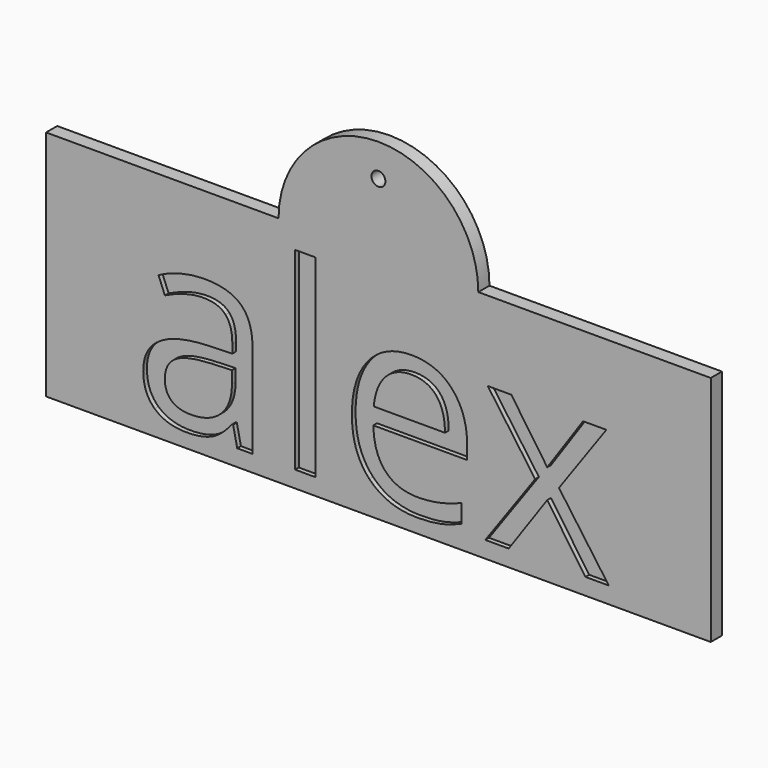
from build123d import *

# Parameters (mm, degrees)
F0_W         = 4.4421075074
F0_H         = 41.6222905751
F0_R         = 1.5
F0_TEXT_SIZE = 54.7774336173
F1_DEPTH     = 2
F2_DEPTH     = 3


# Not quite as in the source:
# - Text() gives the source's letters only with a copy of the font that has no kerning and outlines rounded to 1/6400 em; it was checked with that copy


with BuildPart() as f1:
    # F0 (on Front) → F1 (new body)
    with BuildSketch(Plane.XZ):
        with BuildLine():
            Line((-71.4831541998, -25), (71.4831541998, -25))
            Line((71.4831541998, -25), (71.4831541998, 25))
            Line((71.4831541998, 25), (21.4831541998, 25))
            ThreePointArc((21.4831541998, 25), (0, 46.4831541998), (-21.4831541998, 25))
            Line((-21.4831541998, 25), (-71.4831541998, 25))
            Line((-71.4831541998, 25), (-71.4831541998, -25))
        make_face()
        with BuildLine():
            Line((-27.0763142576, -21.4371655463), (-30.3715192486, -21.4371655463))
            Line((-30.3715192486, -21.4371655463), (-31.2530935709, -17.260386233))
            Line((-31.2530935709, -17.260386233), (-31.4670679209, -17.260386233))
            add(Edge.make_bspline(
                [(-31.4670679209, -17.260386233), (-33.6581652656, -20.0163758618), (-35.8364241493, -20.9963783851)],
                knots=[0, 0, 0, 1, 1, 1], degree=2))
            add(Edge.make_bspline(
                [(-35.8364241493, -20.9963783851), (-38.014683033, -21.9763809085), (-41.284211102, -21.9763809085)],
                knots=[0, 0, 0, 1, 1, 1], degree=2))
            add(Edge.make_bspline(
                [(-41.284211102, -21.9763809085), (-45.6407288694, -21.9763809085), (-48.1142723562, -19.7253707457)],
                knots=[0, 0, 0, 1, 1, 1], degree=2))
            add(Edge.make_bspline(
                [(-48.1142723562, -19.7253707457), (-50.587815843, -17.474360583), (-50.587815843, -13.3318171657)],
                knots=[0, 0, 0, 1, 1, 1], degree=2))
            add(Edge.make_bspline(
                [(-50.587815843, -13.3318171657), (-50.587815843, -4.4561611249), (-36.3884779725, -4.0282124248)],
                knots=[0, 0, 0, 1, 1, 1], degree=2))
            Line((-36.3884779725, -4.0282124248), (-31.4157140769, -3.8655919187))
            Line((-31.4157140769, -3.8655919187), (-31.4157140769, -2.0425304562))
            add(Edge.make_bspline(
                [(-31.4157140769, -2.0425304562), (-31.4157140769, 1.4067360669), (-32.8964165794, 3.0500590754)],
                knots=[0, 0, 0, 1, 1, 1], degree=2))
            add(Edge.make_bspline(
                [(-32.8964165794, 3.0500590754), (-34.3771190819, 4.693382084), (-37.6466471509, 4.693382084)],
                knots=[0, 0, 0, 1, 1, 1], degree=2))
            add(Edge.make_bspline(
                [(-37.6466471509, 4.693382084), (-41.309888024, 4.693382084), (-45.9317339855, 2.4509308953)],
                knots=[0, 0, 0, 1, 1, 1], degree=2))
            Line((-45.9317339855, 2.4509308953), (-47.3011698259, 5.8488435743))
            add(Edge.make_bspline(
                [(-47.3011698259, 5.8488435743), (-45.1357494033, 7.0214230127), (-42.5552187414, 7.6890229849)],
                knots=[0, 0, 0, 1, 1, 1], degree=2))
            add(Edge.make_bspline(
                [(-42.5552187414, 7.6890229849), (-39.9746880796, 8.3566229571), (-37.3727599828, 8.3566229571)],
                knots=[0, 0, 0, 1, 1, 1], degree=2))
            add(Edge.make_bspline(
                [(-37.3727599828, 8.3566229571), (-32.1346678932, 8.3566229571), (-29.6054910754, 6.0328615154)],
                knots=[0, 0, 0, 1, 1, 1], degree=2))
            add(Edge.make_bspline(
                [(-29.6054910754, 6.0328615154), (-27.0763142576, 3.7091000737), (-27.0763142576, -1.426284328)],
                knots=[0, 0, 0, 1, 1, 1], degree=2))
            Line((-27.0763142576, -1.426284328), (-27.0763142576, -21.4371655463))
        make_face(mode=Mode.SUBTRACT)
        with Locations((-15.714276269, -0.6260202587)):
            Rectangle(F0_W, F0_H, mode=Mode.SUBTRACT)
        with BuildLine():
            add(Edge.make_bspline(
                [(13.3733968792, -21.5313142603), (11.2764482486, -21.9763809085), (8.3064842696, -21.9763809085)],
                knots=[0, 0, 0, 1, 1, 1], degree=2))
            add(Edge.make_bspline(
                [(8.3064842696, -21.9763809085), (1.8102230016, -21.9763809085), (-1.9514460726, -18.0135759452)],
                knots=[0, 0, 0, 1, 1, 1], degree=2))
            add(Edge.make_bspline(
                [(-1.9514460726, -18.0135759452), (-5.7131151468, -14.050770982), (-5.7131151468, -7.0238533257)],
                knots=[0, 0, 0, 1, 1, 1], degree=2))
            add(Edge.make_bspline(
                [(-5.7131151468, -7.0238533257), (-5.7131151468, 0.0715361225), (-2.2210537537, 4.2440359488)],
                knots=[0, 0, 0, 1, 1, 1], degree=2))
            add(Edge.make_bspline(
                [(-2.2210537537, 4.2440359488), (1.2710076394, 8.4165357751), (7.1595817533, 8.4165357751)],
                knots=[0, 0, 0, 1, 1, 1], degree=2))
            add(Edge.make_bspline(
                [(7.1595817533, 8.4165357751), (12.663002037, 8.4165357751), (15.872617288, 4.791810285)],
                knots=[0, 0, 0, 1, 1, 1], degree=2))
            add(Edge.make_bspline(
                [(15.872617288, 4.791810285), (19.082232539, 1.1670847949), (19.082232539, -4.772843163)],
                knots=[0, 0, 0, 1, 1, 1], degree=2))
            Line((19.082232539, -4.772843163), (19.082232539, -7.5801866359))
            Line((19.082232539, -7.5801866359), (-1.1083871334, -7.5801866359))
            add(Edge.make_bspline(
                [(-1.1083871334, -7.5801866359), (-0.9714435493, -12.7412479595), (1.5020999375, -15.4159273354)],
                knots=[0, 0, 0, 1, 1, 1], degree=2))
            add(Edge.make_bspline(
                [(1.5020999375, -15.4159273354), (3.9756434243, -18.0906067112), (8.4691047757, -18.0906067112)],
                knots=[0, 0, 0, 1, 1, 1], degree=2))
            add(Edge.make_bspline(
                [(8.4691047757, -18.0906067112), (13.2022173992, -18.0906067112), (17.8240633606, -16.1134837166)],
                knots=[0, 0, 0, 1, 1, 1], degree=2))
            Line((17.8240633606, -16.1134837166), (17.8240633606, -20.0762886799))
            add(Edge.make_bspline(
                [(17.8240633606, -20.0762886799), (15.4703455099, -21.0862476122), (13.3733968792, -21.5313142603)],
                knots=[0, 0, 0, 1, 1, 1], degree=2))
        make_face(mode=Mode.SUBTRACT)
        Polygon((22.9936836583, -21.4371655463), (33.7180780837, -6.4332841195), (23.5243400464, 7.877320413), (28.582693682, 7.877320413), (36.3114472065, -3.3520534786), (44.0145238089, 7.877320413), (49.0215236005, 7.877320413), (38.8277855633, -6.4332841195), (49.5521799887, -21.4371655463), (44.5280622491, -21.4371655463), (36.3114472065, -9.5573096305), (28.0178013979, -21.4371655463), align=None, mode=Mode.SUBTRACT)
        with Locations((0, 39.4689776003)):
            Circle(F0_R, mode=Mode.SUBTRACT)
        with Locations((-53.1041541998, -21.4371655463)):
            Text('alex', F0_TEXT_SIZE, font='Open Sans', text_align=(TextAlign.LEFT, TextAlign.BOTTOM))
        with BuildLine():
            add(Edge.make_bspline(
                [(-44.476708405, -17.0506913699), (-43.0216828246, -18.3045810613), (-40.4026367798, -18.3045810613)],
                knots=[0, 0, 0, 1, 1, 1], degree=2))
            add(Edge.make_bspline(
                [(-40.4026367798, -18.3045810613), (-36.2515343885, -18.3045810613), (-33.8849780767, -16.0321734636)],
                knots=[0, 0, 0, 1, 1, 1], degree=2))
            add(Edge.make_bspline(
                [(-33.8849780767, -16.0321734636), (-31.518421765, -13.7597658659), (-31.518421765, -9.6685762926)],
                knots=[0, 0, 0, 1, 1, 1], degree=2))
            Line((-31.518421765, -9.6685762926), (-31.518421765, -7.0238533257))
            Line((-31.518421765, -7.0238533257), (-35.9605292724, -7.2035917798))
            add(Edge.make_bspline(
                [(-35.9605292724, -7.2035917798), (-41.25853418, -7.3918892079), (-43.5951340828, -8.8511942753)],
                knots=[0, 0, 0, 1, 1, 1], degree=2))
            add(Edge.make_bspline(
                [(-43.5951340828, -8.8511942753), (-45.9317339855, -10.3104993428), (-45.9317339855, -13.3831710097)],
                knots=[0, 0, 0, 1, 1, 1], degree=2))
            add(Edge.make_bspline(
                [(-45.9317339855, -13.3831710097), (-45.9317339855, -15.7968016785), (-44.476708405, -17.0506913699)],
                knots=[0, 0, 0, 1, 1, 1], degree=2))
        make_face()
        with BuildLine():
            add(Edge.make_bspline(
                [(12.4533071739, 2.4594898693), (10.5831713543, 4.693382084), (7.0996689352, 4.693382084)],
                knots=[0, 0, 0, 1, 1, 1], degree=2))
            add(Edge.make_bspline(
                [(7.0996689352, 4.693382084), (3.5733716461, 4.693382084), (1.4721435285, 2.3952975642)],
                knots=[0, 0, 0, 1, 1, 1], degree=2))
            add(Edge.make_bspline(
                [(1.4721435285, 2.3952975642), (-0.6290845892, 0.0972130445), (-1.0056794453, -3.9682996068)],
                knots=[0, 0, 0, 1, 1, 1], degree=2))
            Line((-1.0056794453, -3.9682996068), (14.3234429935, -3.9682996068))
            add(Edge.make_bspline(
                [(14.3234429935, -3.9682996068), (14.3234429935, 0.2255976546), (12.4533071739, 2.4594898693)],
                knots=[0, 0, 0, 1, 1, 1], degree=2))
        make_face()
    extrude(amount=F1_DEPTH)

    # F0 (on Front) → F2 (join)
    with BuildSketch(Plane.XZ):
        with BuildLine():
            Line((-71.4831541998, -25), (71.4831541998, -25))
            Line((71.4831541998, -25), (71.4831541998, 25))
            Line((71.4831541998, 25), (21.4831541998, 25))
            ThreePointArc((21.4831541998, 25), (0, 46.4831541998), (-21.4831541998, 25))
            Line((-21.4831541998, 25), (-71.4831541998, 25))
            Line((-71.4831541998, 25), (-71.4831541998, -25))
        make_face()
        with BuildLine():
            Line((-27.0763142576, -21.4371655463), (-30.3715192486, -21.4371655463))
            Line((-30.3715192486, -21.4371655463), (-31.2530935709, -17.260386233))
            Line((-31.2530935709, -17.260386233), (-31.4670679209, -17.260386233))
            add(Edge.make_bspline(
                [(-31.4670679209, -17.260386233), (-33.6581652656, -20.0163758618), (-35.8364241493, -20.9963783851)],
                knots=[0, 0, 0, 1, 1, 1], degree=2))
            add(Edge.make_bspline(
                [(-35.8364241493, -20.9963783851), (-38.014683033, -21.9763809085), (-41.284211102, -21.9763809085)],
                knots=[0, 0, 0, 1, 1, 1], degree=2))
            add(Edge.make_bspline(
                [(-41.284211102, -21.9763809085), (-45.6407288694, -21.9763809085), (-48.1142723562, -19.7253707457)],
                knots=[0, 0, 0, 1, 1, 1], degree=2))
            add(Edge.make_bspline(
                [(-48.1142723562, -19.7253707457), (-50.587815843, -17.474360583), (-50.587815843, -13.3318171657)],
                knots=[0, 0, 0, 1, 1, 1], degree=2))
            add(Edge.make_bspline(
                [(-50.587815843, -13.3318171657), (-50.587815843, -4.4561611249), (-36.3884779725, -4.0282124248)],
                knots=[0, 0, 0, 1, 1, 1], degree=2))
            Line((-36.3884779725, -4.0282124248), (-31.4157140769, -3.8655919187))
            Line((-31.4157140769, -3.8655919187), (-31.4157140769, -2.0425304562))
            add(Edge.make_bspline(
                [(-31.4157140769, -2.0425304562), (-31.4157140769, 1.4067360669), (-32.8964165794, 3.0500590754)],
                knots=[0, 0, 0, 1, 1, 1], degree=2))
            add(Edge.make_bspline(
                [(-32.8964165794, 3.0500590754), (-34.3771190819, 4.693382084), (-37.6466471509, 4.693382084)],
                knots=[0, 0, 0, 1, 1, 1], degree=2))
            add(Edge.make_bspline(
                [(-37.6466471509, 4.693382084), (-41.309888024, 4.693382084), (-45.9317339855, 2.4509308953)],
                knots=[0, 0, 0, 1, 1, 1], degree=2))
            Line((-45.9317339855, 2.4509308953), (-47.3011698259, 5.8488435743))
            add(Edge.make_bspline(
                [(-47.3011698259, 5.8488435743), (-45.1357494033, 7.0214230127), (-42.5552187414, 7.6890229849)],
                knots=[0, 0, 0, 1, 1, 1], degree=2))
            add(Edge.make_bspline(
                [(-42.5552187414, 7.6890229849), (-39.9746880796, 8.3566229571), (-37.3727599828, 8.3566229571)],
                knots=[0, 0, 0, 1, 1, 1], degree=2))
            add(Edge.make_bspline(
                [(-37.3727599828, 8.3566229571), (-32.1346678932, 8.3566229571), (-29.6054910754, 6.0328615154)],
                knots=[0, 0, 0, 1, 1, 1], degree=2))
            add(Edge.make_bspline(
                [(-29.6054910754, 6.0328615154), (-27.0763142576, 3.7091000737), (-27.0763142576, -1.426284328)],
                knots=[0, 0, 0, 1, 1, 1], degree=2))
            Line((-27.0763142576, -1.426284328), (-27.0763142576, -21.4371655463))
        make_face(mode=Mode.SUBTRACT)
        with Locations((-15.714276269, -0.6260202587)):
            Rectangle(F0_W, F0_H, mode=Mode.SUBTRACT)
        with BuildLine():
            add(Edge.make_bspline(
                [(13.3733968792, -21.5313142603), (11.2764482486, -21.9763809085), (8.3064842696, -21.9763809085)],
                knots=[0, 0, 0, 1, 1, 1], degree=2))
            add(Edge.make_bspline(
                [(8.3064842696, -21.9763809085), (1.8102230016, -21.9763809085), (-1.9514460726, -18.0135759452)],
                knots=[0, 0, 0, 1, 1, 1], degree=2))
            add(Edge.make_bspline(
                [(-1.9514460726, -18.0135759452), (-5.7131151468, -14.050770982), (-5.7131151468, -7.0238533257)],
                knots=[0, 0, 0, 1, 1, 1], degree=2))
            add(Edge.make_bspline(
                [(-5.7131151468, -7.0238533257), (-5.7131151468, 0.0715361225), (-2.2210537537, 4.2440359488)],
                knots=[0, 0, 0, 1, 1, 1], degree=2))
            add(Edge.make_bspline(
                [(-2.2210537537, 4.2440359488), (1.2710076394, 8.4165357751), (7.1595817533, 8.4165357751)],
                knots=[0, 0, 0, 1, 1, 1], degree=2))
            add(Edge.make_bspline(
                [(7.1595817533, 8.4165357751), (12.663002037, 8.4165357751), (15.872617288, 4.791810285)],
                knots=[0, 0, 0, 1, 1, 1], degree=2))
            add(Edge.make_bspline(
                [(15.872617288, 4.791810285), (19.082232539, 1.1670847949), (19.082232539, -4.772843163)],
                knots=[0, 0, 0, 1, 1, 1], degree=2))
            Line((19.082232539, -4.772843163), (19.082232539, -7.5801866359))
            Line((19.082232539, -7.5801866359), (-1.1083871334, -7.5801866359))
            add(Edge.make_bspline(
                [(-1.1083871334, -7.5801866359), (-0.9714435493, -12.7412479595), (1.5020999375, -15.4159273354)],
                knots=[0, 0, 0, 1, 1, 1], degree=2))
            add(Edge.make_bspline(
                [(1.5020999375, -15.4159273354), (3.9756434243, -18.0906067112), (8.4691047757, -18.0906067112)],
                knots=[0, 0, 0, 1, 1, 1], degree=2))
            add(Edge.make_bspline(
                [(8.4691047757, -18.0906067112), (13.2022173992, -18.0906067112), (17.8240633606, -16.1134837166)],
                knots=[0, 0, 0, 1, 1, 1], degree=2))
            Line((17.8240633606, -16.1134837166), (17.8240633606, -20.0762886799))
            add(Edge.make_bspline(
                [(17.8240633606, -20.0762886799), (15.4703455099, -21.0862476122), (13.3733968792, -21.5313142603)],
                knots=[0, 0, 0, 1, 1, 1], degree=2))
        make_face(mode=Mode.SUBTRACT)
        Polygon((22.9936836583, -21.4371655463), (33.7180780837, -6.4332841195), (23.5243400464, 7.877320413), (28.582693682, 7.877320413), (36.3114472065, -3.3520534786), (44.0145238089, 7.877320413), (49.0215236005, 7.877320413), (38.8277855633, -6.4332841195), (49.5521799887, -21.4371655463), (44.5280622491, -21.4371655463), (36.3114472065, -9.5573096305), (28.0178013979, -21.4371655463), align=None, mode=Mode.SUBTRACT)
        with Locations((0, 39.4689776003)):
            Circle(F0_R, mode=Mode.SUBTRACT)
        with BuildLine():
            add(Edge.make_bspline(
                [(12.4533071739, 2.4594898693), (10.5831713543, 4.693382084), (7.0996689352, 4.693382084)],
                knots=[0, 0, 0, 1, 1, 1], degree=2))
            add(Edge.make_bspline(
                [(7.0996689352, 4.693382084), (3.5733716461, 4.693382084), (1.4721435285, 2.3952975642)],
                knots=[0, 0, 0, 1, 1, 1], degree=2))
            add(Edge.make_bspline(
                [(1.4721435285, 2.3952975642), (-0.6290845892, 0.0972130445), (-1.0056794453, -3.9682996068)],
                knots=[0, 0, 0, 1, 1, 1], degree=2))
            Line((-1.0056794453, -3.9682996068), (14.3234429935, -3.9682996068))
            add(Edge.make_bspline(
                [(14.3234429935, -3.9682996068), (14.3234429935, 0.2255976546), (12.4533071739, 2.4594898693)],
                knots=[0, 0, 0, 1, 1, 1], degree=2))
        make_face()
        with BuildLine():
            add(Edge.make_bspline(
                [(-44.476708405, -17.0506913699), (-43.0216828246, -18.3045810613), (-40.4026367798, -18.3045810613)],
                knots=[0, 0, 0, 1, 1, 1], degree=2))
            add(Edge.make_bspline(
                [(-40.4026367798, -18.3045810613), (-36.2515343885, -18.3045810613), (-33.8849780767, -16.0321734636)],
                knots=[0, 0, 0, 1, 1, 1], degree=2))
            add(Edge.make_bspline(
                [(-33.8849780767, -16.0321734636), (-31.518421765, -13.7597658659), (-31.518421765, -9.6685762926)],
                knots=[0, 0, 0, 1, 1, 1], degree=2))
            Line((-31.518421765, -9.6685762926), (-31.518421765, -7.0238533257))
            Line((-31.518421765, -7.0238533257), (-35.9605292724, -7.2035917798))
            add(Edge.make_bspline(
                [(-35.9605292724, -7.2035917798), (-41.25853418, -7.3918892079), (-43.5951340828, -8.8511942753)],
                knots=[0, 0, 0, 1, 1, 1], degree=2))
            add(Edge.make_bspline(
                [(-43.5951340828, -8.8511942753), (-45.9317339855, -10.3104993428), (-45.9317339855, -13.3831710097)],
                knots=[0, 0, 0, 1, 1, 1], degree=2))
            add(Edge.make_bspline(
                [(-45.9317339855, -13.3831710097), (-45.9317339855, -15.7968016785), (-44.476708405, -17.0506913699)],
                knots=[0, 0, 0, 1, 1, 1], degree=2))
        make_face()
    extrude(amount=F2_DEPTH)


solid = f1.part
